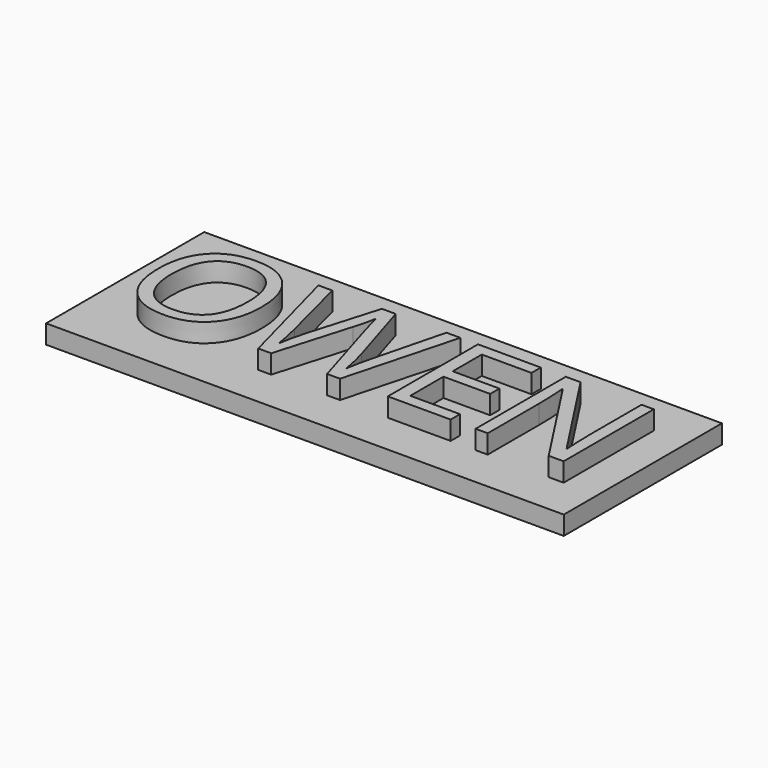
from build123d import *

# Parameters (mm, degrees)
F0_W         = 110
F0_H         = 42
F1_DEPTH     = 4
F2_TEXT_SIZE = 33.5429769392
F3_DEPTH     = 4


# Not quite as in the source:
# - Text() gives the source's letters only with a copy of the font that has no kerning and outlines rounded to 1/6400 em; it was checked with that copy


with BuildPart() as f1:
    # F0 (on Top) → F1 (new body)
    with BuildSketch(Plane.XY):
        Rectangle(F0_W, F0_H)
    extrude(amount=F1_DEPTH)

    # F2 (on face) → F3 (join)
    with BuildSketch(Plane.XY.offset(4)):
        with Locations((-50, -12.0709433962)):
            Text('OWEN', F2_TEXT_SIZE, font='Open Sans', text_align=(TextAlign.LEFT, TextAlign.BOTTOM))
    extrude(amount=F3_DEPTH)


solid = f1.part
